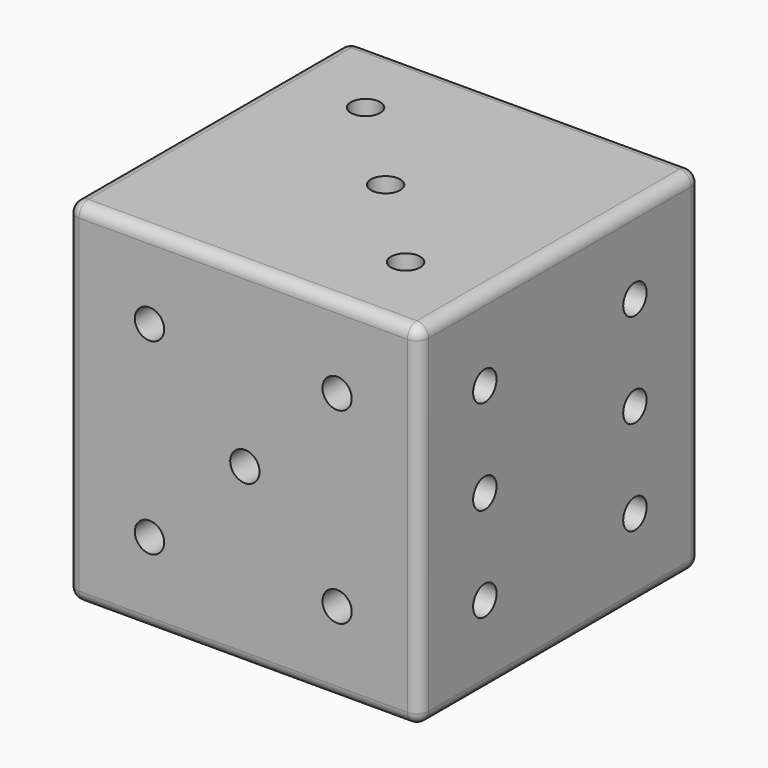
from build123d import *

# Parameters (mm, degrees)
F1_DEPTH     = 15
F2_R         = 1
F3_T1_DEPTH  = 28
F3_S5_W      = 1
F3_S5_H      = 1
F3_T6_DEPTH  = 1
F3_S11_W     = 1
F3_S11_H     = 1
F3_T12_DEPTH = 1
F10_D        = 2.5
F10_DEPTH    = 3
F10_TIP      = 0.7510757738
F11_D        = 2.5
F11_DEPTH    = 3
F11_TIP      = 0.7510757738
F12_D        = 2.5
F12_DEPTH    = 3
F12_TIP      = 0.7510757738
F13_D        = 2.5
F13_DEPTH    = 3
F13_TIP      = 0.7510757738
F14_D        = 2.5
F14_DEPTH    = 3
F14_TIP      = 0.7510757738
F15_D        = 2.5
F15_DEPTH    = 3
F15_TIP      = 0.7510757738


# Not quite as in the source:
# - a fillet or chamfer that OpenCascade refuses, or shapes differently, is made with other operations: its cross-section is extruded or revolved along the edge and cut away or added


with BuildPart() as f1:
    # F0 (on Front) → F1 (new body, symmetric)
    with BuildSketch(Plane.XZ):
        Polygon((-0.1339098811, 0.0507837534), (-15.1339098811, 15.0507837534), (-15.1339098811, -14.9492162466), align=None)
        Polygon((14.8660901189, 15.0507837534), (-15.1339098811, 15.0507837534), (-0.1339098811, 0.0507837534), align=None)
        Polygon((14.8660901189, -14.9492162466), (14.8660901189, 15.0507837534), (-0.1339098811, 0.0507837534), align=None)
        Polygon((-0.1339098811, 0.0507837534), (-15.1339098811, -14.9492162466), (14.8660901189, -14.9492162466), align=None)
    extrude(amount=F1_DEPTH, both=True)

    # F2
    f2_edges = [f1.edges().sort_by_distance(p)[0] for p in [
        (-0.13391, -15, 15.050784),
        (14.86609, 0, 15.050784),
        (-0.13391, 15, 15.050784),
        (-15.13391, 0, 15.050784),
        (-15.13391, 15, 0.050784),
        (14.86609, 15, 0.050784),
        (14.86609, -15, 0.050784),
        (-0.13391, -15, -14.949216),
        (14.86609, 0, -14.949216),
        (-15.13391, 0, -14.949216),
        (-0.13391, 15, -14.949216),
    ]]
    fillet(f2_edges, radius=F2_R)

    # F3: fillet of radius 1 on 1 edges, made by hand

    # F3_s2 → F3_t1 (cut)
    with BuildSketch(Plane.XY.offset(-13.9492162466)):
        with BuildLine():
            ThreePointArc((-15.1339098811, -14), (-14.8410166623, -14.7071067812), (-14.1339098811, -15))
            Line((-14.1339098811, -15), (-15.1339098811, -15))
            Line((-15.1339098811, -15), (-15.1339098811, -14))
        make_face()
    extrude(amount=F3_T1_DEPTH, mode=Mode.SUBTRACT)


with BuildPart() as f3_tool4:
    # F3_s5 → F3_t6 (new body)
    with BuildSketch(Plane.YZ.offset(-14.1339098811)):
        with Locations((-14.5, 14.5507837534)):
            Rectangle(F3_S5_W, F3_S5_H)
    extrude(amount=-F3_T6_DEPTH)

    # F3_s7 → F3_t8 (revolve, cut)
    with BuildSketch(Plane(origin=(-14.1339098811, -14, 14.0507837534), x_dir=(0, 0.7071067812, -0.7071067812), z_dir=(0, 0.7071067812, 0.7071067812))):
        with BuildLine():
            ThreePointArc((0, -1), (1, 0), (0, 1))
            Line((0, 1), (0, -1))
        make_face()
    revolve(axis=Axis((-14.1339098811, -14, 14.0507837534), (-1, 0, 0)), mode=Mode.SUBTRACT)


with BuildPart() as f1_1:
    add(f1.part)

    # F3_t3: cut F3_tool4
    add(f3_tool4.part, mode=Mode.SUBTRACT)


with BuildPart() as f3_tool10:
    # F3_s11 → F3_t12 (new body)
    with BuildSketch(Plane.YZ.offset(-14.1339098811)):
        with Locations((-14.5, -14.4492162466)):
            Rectangle(F3_S11_W, F3_S11_H)
    extrude(amount=-F3_T12_DEPTH)

    # F3_s13 → F3_t14 (revolve, cut)
    with BuildSketch(Plane(origin=(-14.1339098811, -14, -13.9492162466), x_dir=(0, 0.7071067812, 0.7071067812), z_dir=(0, -0.7071067812, 0.7071067812))):
        with BuildLine():
            ThreePointArc((0, -1), (1, 0), (0, 1))
            Line((0, 1), (0, -1))
        make_face()
    revolve(axis=Axis((-14.1339098811, -14, -13.9492162466), (-1, 0, 0)), mode=Mode.SUBTRACT)


with BuildPart() as f1_2:
    add(f1_1.part)

    # F3_t9: cut F3_tool10
    add(f3_tool10.part, mode=Mode.SUBTRACT)

    # F10
    with Locations(Plane(origin=(-15.1339098811, 0, 0), x_dir=(0, -1, 0), z_dir=(-1, 0, 0))):
        with Locations((0, 0)):
            Hole(F10_D / 2, depth=F10_DEPTH)
            with Locations((0, 0, -(F10_DEPTH + F10_TIP / 2))):  # 118° drill point
                Cone(0, F10_D / 2, F10_TIP, mode=Mode.SUBTRACT)

    # F11
    with Locations(Plane(origin=(0, 15, 0), x_dir=(-1, 0, 0), z_dir=(0, 1, 0))):
        with Locations((8.0831261277, 8), (-8.0831261277, -8)):
            Hole(F11_D / 2, depth=F11_DEPTH)
            with Locations((0, 0, -(F11_DEPTH + F11_TIP / 2))):  # 118° drill point
                Cone(0, F11_D / 2, F11_TIP, mode=Mode.SUBTRACT)

    # F12
    with Locations(Plane.XY.offset(15.0507837534)):
        with Locations((-8, 7.8672532922), (0, 0), (8, -7.8672532922)):
            Hole(F12_D / 2, depth=F12_DEPTH)
            with Locations((0, 0, -(F12_DEPTH + F12_TIP / 2))):  # 118° drill point
                Cone(0, F12_D / 2, F12_TIP, mode=Mode.SUBTRACT)

    # F13
    with Locations(Plane(origin=(0, 0, -14.9492162466), x_dir=(1, 0, 0), z_dir=(0, 0, -1))):
        with Locations((-8, 7.8660901189), (8, 7.8660901189), (8, -7.8660901189), (-8, -7.8660901189)):
            Hole(F13_D / 2, depth=F13_DEPTH)
            with Locations((0, 0, -(F13_DEPTH + F13_TIP / 2))):  # 118° drill point
                Cone(0, F13_D / 2, F13_TIP, mode=Mode.SUBTRACT)

    # F14
    with Locations(Plane.YZ.offset(14.8660901189)):
        with Locations((-8, 8.0507837534), (-8, 0), (-8, -8.0507837534), (8, -8.0507837534), (8, 0), (8, 8.0507837534)):
            Hole(F14_D / 2, depth=F14_DEPTH)
            with Locations((0, 0, -(F14_DEPTH + F14_TIP / 2))):  # 118° drill point
                Cone(0, F14_D / 2, F14_TIP, mode=Mode.SUBTRACT)

    # F15
    with Locations(Plane.XZ.offset(15)):
        with Locations((-8.1339098811, 8.0507837534), (0, 0), (7.8660901189, 8.0507837534), (7.8660901189, -7.9492162466), (-8.1339098811, -7.9492162466)):
            Hole(F15_D / 2, depth=F15_DEPTH)
            with Locations((0, 0, -(F15_DEPTH + F15_TIP / 2))):  # 118° drill point
                Cone(0, F15_D / 2, F15_TIP, mode=Mode.SUBTRACT)


solid = f1_2.part
